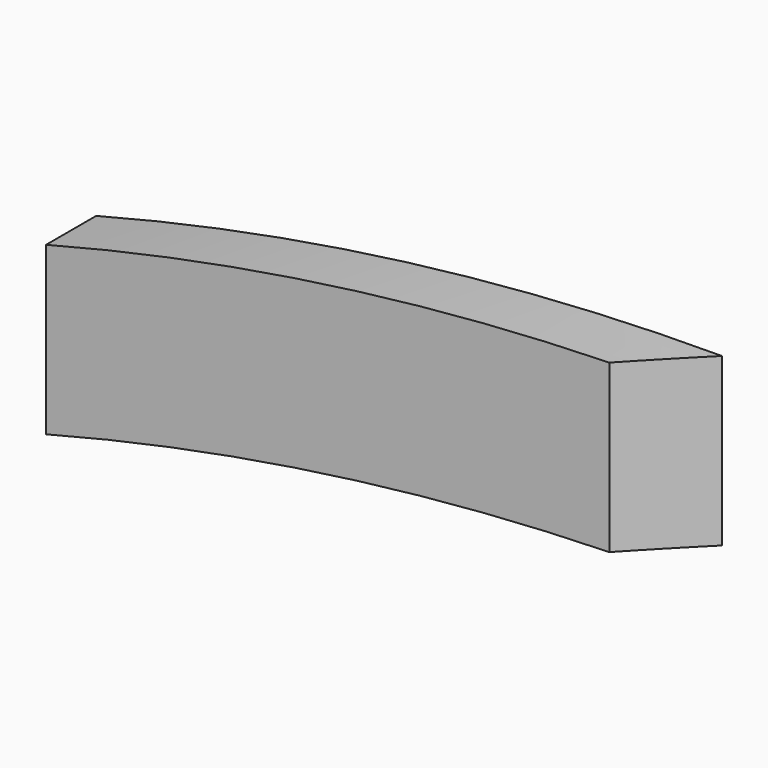
from build123d import *

# Parameters (mm, degrees)
F1_DEPTH = 7.5
F2_SIZE  = 7.49999


# Not quite as in the source:
# - a fillet or chamfer is up to 0.001 mm smaller than in the source, because OpenCascade refuses the exact size


with BuildPart() as f1:
    # F0 (on Front) → F1 (new body)
    with BuildSketch(Plane.XZ):
        with BuildLine():
            Line((-86.7414106019, 13.5850626232), (-86.7414106019, -6.4149373768))
            ThreePointArc((-86.7414106019, -6.4149373768), (-49.5427734858, 0.7956791903), (-11.7279719579, 3.1982569702))
            Line((-11.7279719579, 3.1982569702), (-11.7279719579, 23.1982569702))
            ThreePointArc((-11.7279719579, 23.1982569702), (-49.5427734858, 20.7956791903), (-86.7414106019, 13.5850626232))
        make_face()
    extrude(amount=F1_DEPTH)

    # F2 (size 7.5 in the source; OpenCascade refuses exactly that, so slightly less here)
    f2_edges = [f1.edges().sort_by_distance(p)[0] for p in [
        (-11.727972, -7.5, 13.198257),
    ]]
    chamfer(f2_edges, length=F2_SIZE)


solid = f1.part
